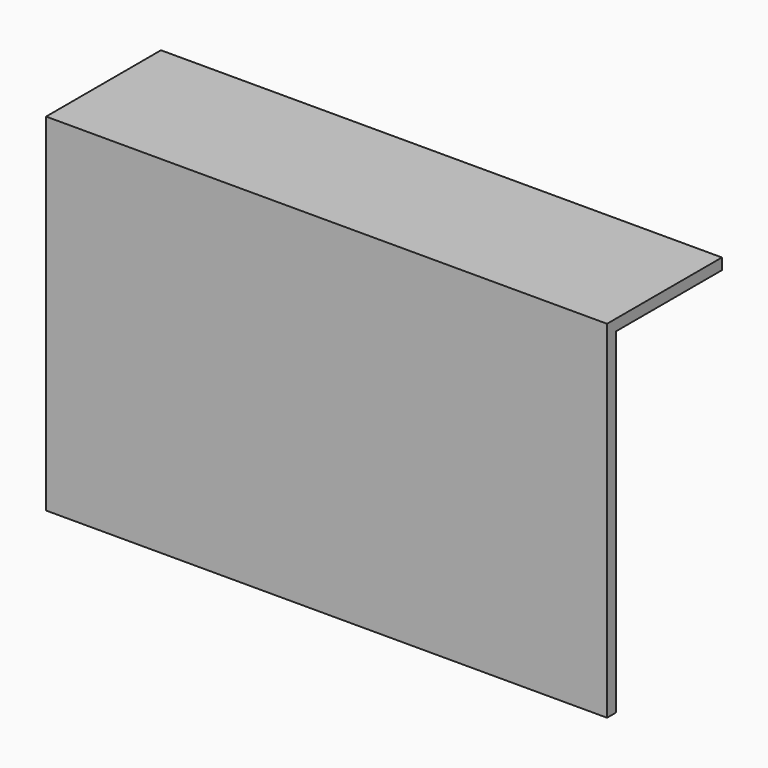
from build123d import *

# Parameters (mm, degrees)
F0_W     = 127
F0_H     = 78.5267129702
F1_DEPTH = 32.512
F2_T     = -2.54


# Not quite as in the source:
# - a feature of the source that left no trace in its solid (it failed there, or was rolled back) is left out


with BuildPart() as f1:
    # F0 (on Front) → F1 (new body)
    with BuildSketch(Plane.XZ):
        with Locations((-42.0160433277, -23.7329155207)):
            Rectangle(F0_W, F0_H)
    extrude(amount=F1_DEPTH)

    # F2
    f2_openings = [f1.faces().sort_by_distance(p)[0] for p in [
        (21.483957, -16.256, -23.732916),
        (-42.016043, -16.256, -62.996272),
        (-42.016043, 0, -23.732916),
    ]]
    offset(amount=F2_T, openings=f2_openings)


solid = f1.part
